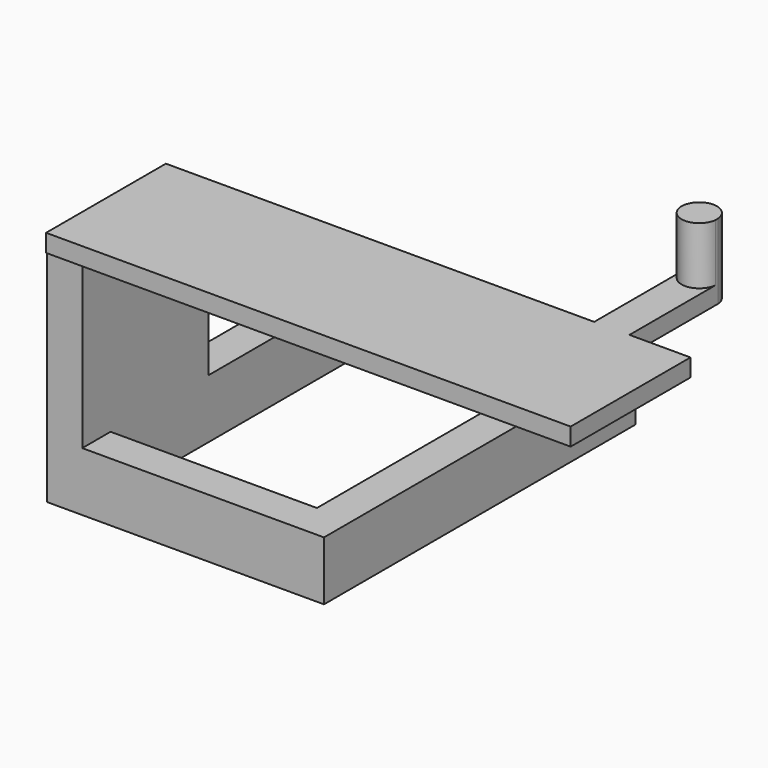
from build123d import *

# Parameters (mm, degrees)
F1_DEPTH      = 5
F2_DEPTH      = 19.05
F3_DEPTH      = 5
F4_W          = 12.7
F4_H          = 1.5
F5_DEPTH      = 37.23736246
F5_DEPTH_BACK = 7.25
F6_START      = 18.6339281499
F6_DEPTH      = 1.5
F7_START      = 18.6339281499
F7_DEPTH      = 6.3660718501


with BuildPart() as f1:
    # F0 (on Top) → F1 (new body)
    with BuildSketch(Plane.XY):
        Polygon((-34.23736246, 9.9433793599), (-34.23736246, 6.9433793599), (-16.73736246, 6.9433793599), (-16.73736246, -20.0566206401), (-34.23736246, -20.0566206401), (-34.23736246, -23.0566206401), (-13.73736246, -23.0566206401), (-13.73736246, 9.9433793599), align=None)
    extrude(amount=F1_DEPTH)

    # F0 (on Top) → F2 (join)
    with BuildSketch(Plane.XY):
        Polygon((-34.23736246, -20.0566206401), (-34.23736246, -9.6503041635), (-37.23736246, -9.6503041635), (-37.23736246, -23.0566206401), (-34.23736246, -23.0566206401), align=None)
    extrude(amount=F2_DEPTH)

    # F0 (on Top) → F3 (join)
    with BuildSketch(Plane.XY):
        Polygon((-34.23736246, -9.6503041635), (-34.23736246, 6.9433793599), (-34.23736246, 9.9433793599), (-37.23736246, 9.9433793599), (-37.23736246, -9.6503041635), align=None)
    extrude(amount=F3_DEPTH)

    # F4 (on Right) → F5 (join, two sides)
    with BuildSketch(Plane.YZ) as f5_sk:
        with Locations((-16.7916113675, 19.3839281499)):
            Rectangle(F4_W, F4_H)
    extrude(amount=-F5_DEPTH)
    extrude(f5_sk.sketch, amount=F5_DEPTH_BACK)

    # F0 (on Top) → F6 (join)
    with BuildSketch(Plane.XY.offset(F6_START)):
        with BuildLine():
            Line((2.0767554697, -8.3933884358), (2.0767554697, -1.3145332665))
            ThreePointArc((2.0767554697, -1.3145332665), (0.5588870059, -2.6728853277), (-0.9137062697, -1.2655779555))
            Line((-0.9137062697, -1.2655779555), (-0.9137062697, -8.3933884358))
            Line((-0.9137062697, -8.3933884358), (-0.9137062697, -23.0566206401))
            Line((-0.9137062697, -23.0566206401), (2.0767554697, -23.0566206401))
            Line((2.0767554697, -23.0566206401), (2.0767554697, -8.3933884358))
        make_face()
    extrude(amount=F6_DEPTH)

    # F0 (on Top) → F7 (join)
    with BuildSketch(Plane.XY.offset(F7_START)):
        with BuildLine():
            Line((2.0767554697, -1.3145332665), (2.0767554697, -1.0316392973))
            ThreePointArc((2.0767554697, -1.0316392973), (0.5588870059, 0.3267127639), (-0.9137062697, -1.0805946084))
            Line((-0.9137062697, -1.0805946084), (-0.9137062697, -1.2655779555))
            ThreePointArc((-0.9137062697, -1.2655779555), (0.5588870059, -2.6728853277), (2.0767554697, -1.3145332665))
        make_face()
    extrude(amount=F7_DEPTH)


solid = f1.part
